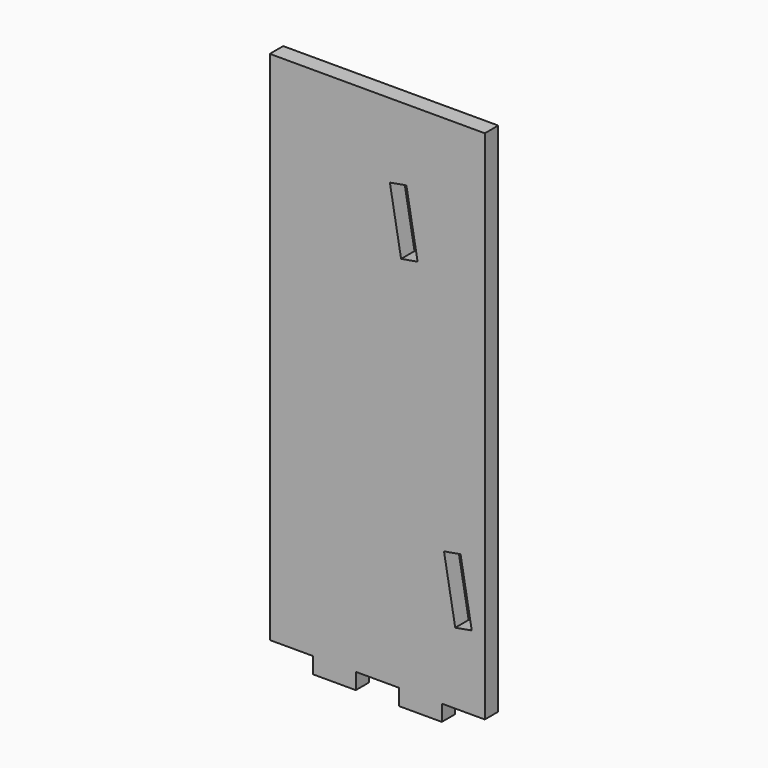
from build123d import *

# Parameters (mm, degrees)
F0_W     = 50.8
F0_H     = 19.05
F1_DEPTH = 19.812


# Not quite as in the source:
# - a feature names something its author has since deleted; it is built from what else it names


with BuildPart() as f1:
    # F0 (on Front) → F1 (new body)
    with BuildSketch(Plane.XZ):
        Polygon((239.4815002712, 559.237990855), (-14.5184997288, 559.237990855), (-14.5184997288, -50.362009145), (36.2815002712, -50.362009145), (87.0815002712, -50.362009145), (137.8815002712, -50.362009145), (188.6815002712, -50.362009145), (219.3638682365, -50.362009145), (204.533166074, 33.7470824019), (191.3011749357, 108.7894331814), (140.5785422392, 396.4517778362), (127.346551101, 471.4941286158), (113.5079391308, 549.9767970912), (133.6255711655, 549.9767970912), (146.8575623037, 474.9344463117), (160.0895534419, 399.8920955322), (210.8121861384, 112.2297508773), (224.0441772766, 37.1874000978), (239.4815002712, -50.362009145), align=None)
        with Locations((61.6815002712, -59.887009145)):
            Rectangle(F0_W, F0_H)
        with Locations((163.2815002712, -59.887009145)):
            Rectangle(F0_W, F0_H)
        Polygon((127.346551101, 471.4941286158), (146.8575623037, 474.9344463117), (133.6255711655, 549.9767970912), (113.5079391308, 549.9767970912), align=None)
        Polygon((219.3638682365, -50.362009145), (239.4815002712, -50.362009145), (224.0441772766, 37.1874000978), (204.533166074, 33.7470824019), align=None)
        Polygon((191.3011749357, 108.7894331814), (210.8121861384, 112.2297508773), (160.0895534419, 399.8920955322), (140.5785422392, 396.4517778362), align=None)
    extrude(amount=F1_DEPTH)


solid = f1.part
